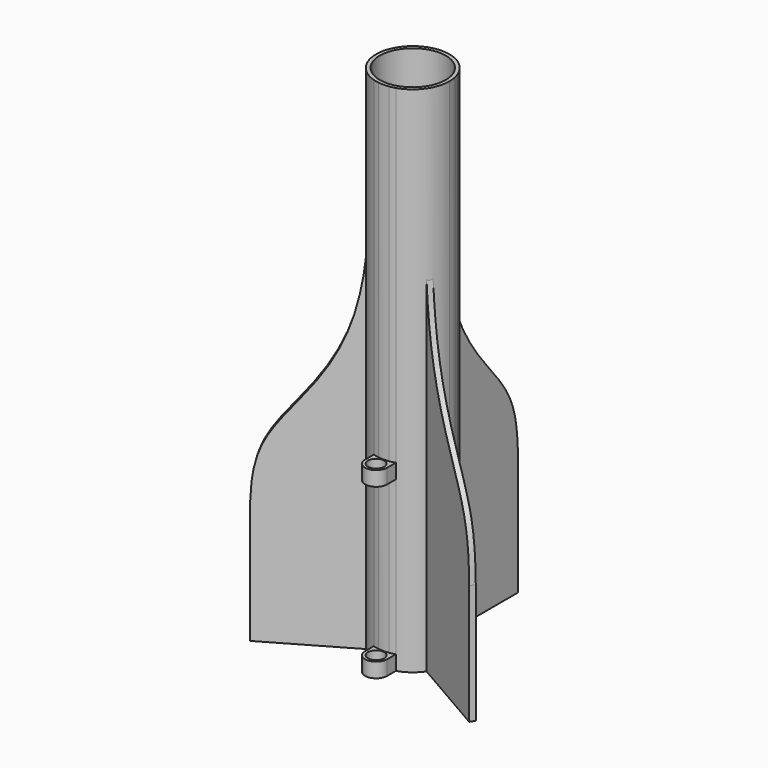
from build123d import *

# Parameters (mm, degrees)
F0_R     = 9
F1_DEPTH = 140
F2_DEPTH = 100
F4_DEPTH = 10.751
F5_COUNT = 3
F0_R_2   = 2.25
F6_DEPTH = 4
F7_START = 46
F7_DEPTH = 4
F8_START = 62
F0_R_3   = 7.5
F8_DEPTH = 3


# Not quite as in the source:
# - a feature names something its author has since deleted; it is built from what else it names


with BuildPart() as f1:
    # F0 (on Top) → F1 (new body)
    with BuildSketch(Plane.XY):
        with BuildLine():
            ThreePointArc((-3, -9.5393920142), (-2.2464281062, -9.744411771), (-1.4791551643, -9.89))
            ThreePointArc((-1.4791551643, -9.89), (0, -10), (1.4791551643, -9.89))
            ThreePointArc((1.4791551643, -9.89), (2.2464281062, -9.744411771), (3, -9.5393920142))
            ThreePointArc((3, -9.5393920142), (8.0622577483, -5.9160797831), (10, 0))
            ThreePointArc((10, 0), (7.3314391493, 6.8007352544), (0.75, 9.9718353376))
            ThreePointArc((0.75, 9.9718353376), (0, 10), (-0.75, 9.9718353376))
            ThreePointArc((-0.75, 9.9718353376), (-9.9341644436, 1.1455901566), (-3, -9.5393920142))
        make_face()
        Circle(F0_R, mode=Mode.SUBTRACT)
    extrude(amount=F1_DEPTH)

    # F0 (on Top) → F2 (join)
    with BuildSketch(Plane.XY):
        with BuildLine():
            Line((-0.75, 34.9718353376), (-0.75, 9.9718353376))
            ThreePointArc((-0.75, 9.9718353376), (0, 10), (0.75, 9.9718353376))
            Line((0.75, 9.9718353376), (0.75, 34.9718353376))
            Line((0.75, 34.9718353376), (-0.75, 34.9718353376))
        make_face()
    extrude(amount=F2_DEPTH)

    # F3 (on face) → F4 (cut, through all)
    with BuildSketch(Plane.YZ.offset(0.75)):
        with BuildLine():
            Line((34.9718353376, 100), (9.9718353376, 100))
            Line((9.9718353376, 100), (9.9718353376, 94.1647440576))
            add(Edge.make_bspline(
                [(9.9718353376, 94.1647440576), (10.1832449594, 91.2204140215), (12.0836351221, 77.2918027042), (20.9708053433, 61.8272021249), (33.801245613, 48.6414831262), (34.7842815391, 38.599508776), (34.9718353376, 32.702038365)],
                knots=[0.0899218527, 0.0899218527, 0.0899218527, 0.0899218527, 0.2371904705, 0.3995520788, 0.5544857931, 0.7015059428, 0.7015059428, 0.7015059428, 0.7015059428], degree=3))
            Line((34.9718353376, 32.702038365), (34.9718353376, 100))
        make_face()
    extrude(amount=-F4_DEPTH, mode=Mode.SUBTRACT)


with BuildPart() as f5_1:
    # F5: instance of F1
    add(f1.part.rotate(Axis((0, 0, 0), (0, 0, 1)), 1 * 360 / F5_COUNT))


with BuildPart() as f5_2:
    # F5: instance of F1
    add(f1.part.rotate(Axis((0, 0, 0), (0, 0, 1)), 2 * 360 / F5_COUNT))


with BuildPart() as f1_1:
    add(f1.part)

    add(f5_1.part)  # F6 merges F5_1

    add(f5_2.part)  # F6 merges F5_2
    # F0 (on Top) → F6 (join)
    with BuildSketch(Plane.XY):
        with BuildLine():
            ThreePointArc((1.4791551643, -9.89), (0, -10), (-1.4791551643, -9.89))
            ThreePointArc((-1.4791551643, -9.89), (-2.592051841, -10.9896135416), (-3, -12.5))
            ThreePointArc((-3, -12.5), (0, -15.5), (3, -12.5))
            ThreePointArc((3, -12.5), (2.592051841, -10.9896135416), (1.4791551643, -9.89))
        make_face()
        with Locations((0, -12.5)):
            Circle(F0_R_2, mode=Mode.SUBTRACT)
        with BuildLine():
            ThreePointArc((-3, -12.5), (-2.592051841, -10.9896135416), (-1.4791551643, -9.89))
            ThreePointArc((-1.4791551643, -9.89), (-2.2464281062, -9.744411771), (-3, -9.5393920142))
            Line((-3, -9.5393920142), (-3, -12.5))
        make_face()
        with BuildLine():
            ThreePointArc((3, -9.5393920142), (2.2464281062, -9.744411771), (1.4791551643, -9.89))
            ThreePointArc((1.4791551643, -9.89), (2.592051841, -10.9896135416), (3, -12.5))
            Line((3, -12.5), (3, -9.5393920142))
        make_face()
    extrude(amount=F6_DEPTH)

    # F0 (on Top) → F7 (join)
    with BuildSketch(Plane.XY.offset(F7_START)):
        with BuildLine():
            ThreePointArc((1.4791551643, -9.89), (0, -10), (-1.4791551643, -9.89))
            ThreePointArc((-1.4791551643, -9.89), (-2.592051841, -10.9896135416), (-3, -12.5))
            ThreePointArc((-3, -12.5), (0, -15.5), (3, -12.5))
            ThreePointArc((3, -12.5), (2.592051841, -10.9896135416), (1.4791551643, -9.89))
        make_face()
        with Locations((0, -12.5)):
            Circle(F0_R_2, mode=Mode.SUBTRACT)
        with BuildLine():
            ThreePointArc((-3, -12.5), (-2.592051841, -10.9896135416), (-1.4791551643, -9.89))
            ThreePointArc((-1.4791551643, -9.89), (-2.2464281062, -9.744411771), (-3, -9.5393920142))
            Line((-3, -9.5393920142), (-3, -12.5))
        make_face()
        with BuildLine():
            ThreePointArc((3, -9.5393920142), (2.2464281062, -9.744411771), (1.4791551643, -9.89))
            ThreePointArc((1.4791551643, -9.89), (2.592051841, -10.9896135416), (3, -12.5))
            Line((3, -12.5), (3, -9.5393920142))
        make_face()
    extrude(amount=F7_DEPTH)

    # F0 (on Top) → F8 (join)
    with BuildSketch(Plane.XY.offset(F8_START)):
        Circle(F0_R)
        Circle(F0_R_3, mode=Mode.SUBTRACT)
    extrude(amount=F8_DEPTH)


solid = f1_1.part
